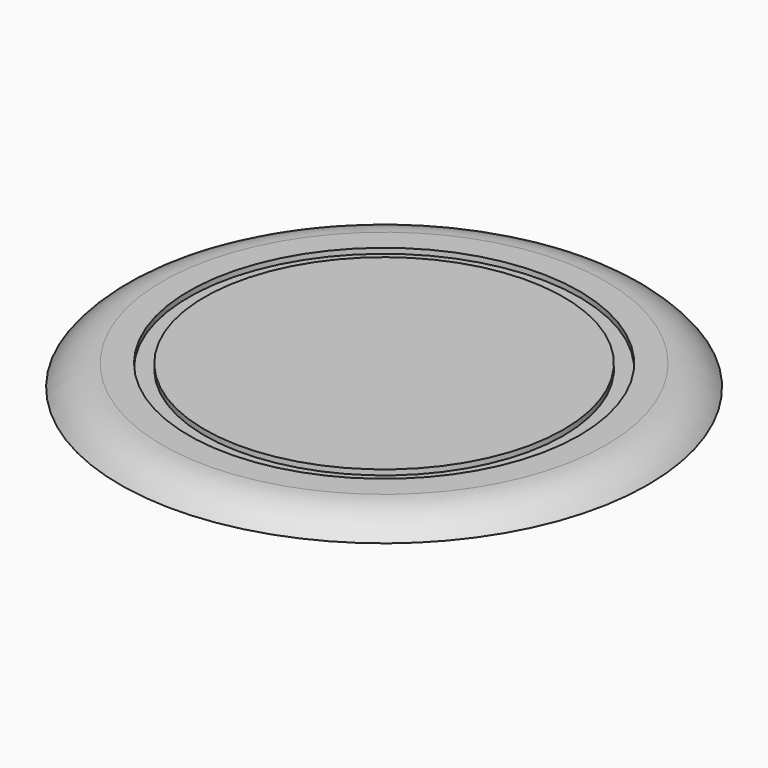
from build123d import *

# Parameters (mm, degrees)
F0_R     = 50
F1_DEPTH = 4
F3_R     = 37
F3_R_2   = 34
F4_DEPTH = 1


# Not quite as in the source:
# - a fillet or chamfer that OpenCascade refuses, or shapes differently, is made with other operations: its cross-section is extruded or revolved along the edge and cut away or added


with BuildPart() as f1:
    # F0 (on Top) → F1 (new body)
    with BuildSketch(Plane.XY):
        Circle(F0_R)
    extrude(amount=F1_DEPTH)

    # F2: fillet of radius 10 on 1 edges, made by hand

    # F2_s1 → F2_t2 (revolve, cut)
    with BuildSketch(Plane.XZ):
        with BuildLine():
            ThreePointArc((50, 0), (46.472135955, 2.94427191), (42, 4))
            Line((42, 4), (50, 4))
            Line((50, 4), (50, 0))
        make_face()
    revolve(axis=Axis((0, 0, 4), (0, 0, 1)), mode=Mode.SUBTRACT)

    # F3 (on face) → F4 (cut)
    with BuildSketch(Plane.XY.offset(4)):
        Circle(F3_R)
        Circle(F3_R_2, mode=Mode.SUBTRACT)
    extrude(amount=-F4_DEPTH, mode=Mode.SUBTRACT)


solid = f1.part
